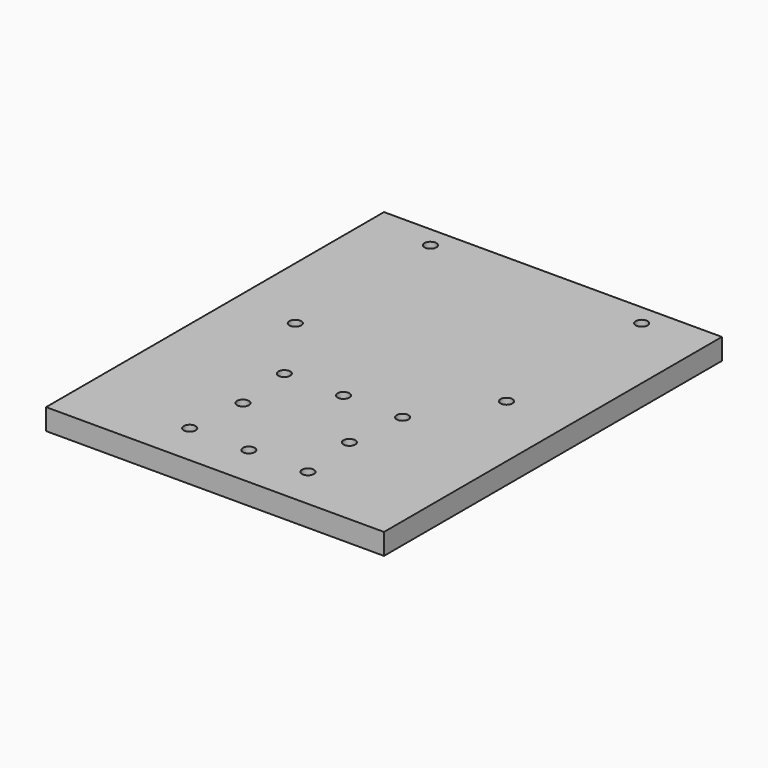
from build123d import *

# Parameters (mm, degrees)
F0_W     = 101.6
F0_H     = 127
F0_R     = 1.778
F1_DEPTH = 6.35


# Not quite as in the source:
# - a length typed as a fraction of an inch, garbled in the dataset ("3 / 203.2 mm" for 3/8 in), is restored


with BuildPart() as f1:
    # F0 (on Top) → F1 (new body)
    with BuildSketch(Plane.XY):
        with Locations((50.8, 63.5)):
            Rectangle(F0_W, F0_H)
        with Locations((33.022, 12.7)):
            Circle(F0_R, mode=Mode.SUBTRACT)
        with Locations((50.8, 12.7)):
            Circle(F0_R, mode=Mode.SUBTRACT)
        with Locations((34.8, 30.478)):
            Circle(F0_R, mode=Mode.SUBTRACT)
        with Locations((33.022, 48.256)):
            Circle(F0_R, mode=Mode.SUBTRACT)
        with Locations((50.8, 48.256)):
            Circle(F0_R, mode=Mode.SUBTRACT)
        with Locations((68.578, 12.7)):
            Circle(F0_R, mode=Mode.SUBTRACT)
        with Locations((66.8, 30.478)):
            Circle(F0_R, mode=Mode.SUBTRACT)
        with Locations((68.578, 48.256)):
            Circle(F0_R, mode=Mode.SUBTRACT)
        with Locations((19.05, 69.85)):
            Circle(F0_R, mode=Mode.SUBTRACT)
        with Locations((19.05, 120.65)):
            Circle(F0_R, mode=Mode.SUBTRACT)
        with Locations((82.55, 69.85)):
            Circle(F0_R, mode=Mode.SUBTRACT)
        with Locations((82.55, 120.65)):
            Circle(F0_R, mode=Mode.SUBTRACT)
    extrude(amount=F1_DEPTH)


solid = f1.part
